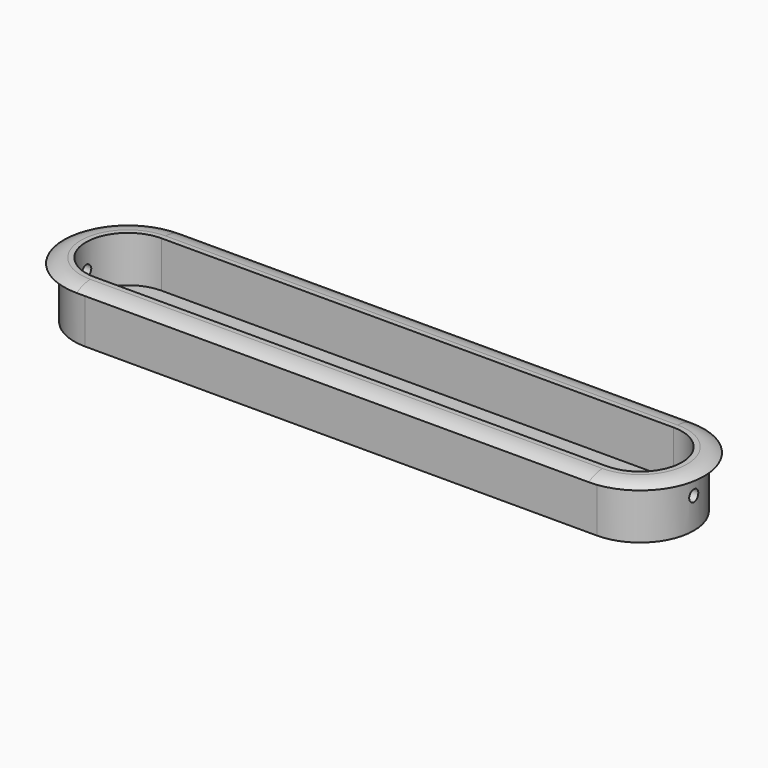
from build123d import *

# Parameters (mm, degrees)
F1_DEPTH    = 10
F3_DEPTH    = 1
F4_T1_DEPTH = 100
F4_T4_ANGLE = 180
F4_T6_ANGLE = 180
F6_DEPTH    = 9
F7_R        = 1.1168399156
F8_DEPTH    = 100


# Not quite as in the source:
# - a fillet or chamfer that OpenCascade refuses, or shapes differently, is made with other operations: its cross-section is extruded or revolved along the edge and cut away or added


with BuildPart() as f1:
    # F0 (on Top) → F1 (new body)
    with BuildSketch(Plane.XY):
        with BuildLine():
            Line((48.6515399069, 4.7592671573), (-51.3484600931, 4.7592671573))
            ThreePointArc((-51.3484600931, 4.7592671573), (-61.8484600931, -5.7407328427), (-51.3484600931, -16.2407328427))
            Line((-51.3484600931, -16.2407328427), (48.6515399069, -16.2407328427))
            ThreePointArc((48.6515399069, -16.2407328427), (59.1515399069, -5.7407328427), (48.6515399069, 4.7592671573))
        make_face()
    extrude(amount=F1_DEPTH)

    # F2 (on face) → F3 (join)
    with BuildSketch(Plane.XY.offset(10)):
        with BuildLine():
            Line((48.6515399069, 6.7592671573), (-51.3484600931, 6.7592671573))
            ThreePointArc((-51.3484600931, 6.7592671573), (-63.8484600931, -5.7407328427), (-51.3484600931, -18.2407328427))
            Line((-51.3484600931, -18.2407328427), (48.6515399069, -18.2407328427))
            ThreePointArc((48.6515399069, -18.2407328427), (61.1515399069, -5.7407328427), (48.6515399069, 6.7592671573))
        make_face()
        with BuildLine():
            Line((-51.3484600931, 4.7592671573), (48.6515399069, 4.7592671573))
            ThreePointArc((48.6515399069, 4.7592671573), (59.1515399069, -5.7407328427), (48.6515399069, -16.2407328427))
            Line((48.6515399069, -16.2407328427), (-51.3484600931, -16.2407328427))
            ThreePointArc((-51.3484600931, -16.2407328427), (-61.8484600931, -5.7407328427), (-51.3484600931, 4.7592671573))
        make_face(mode=Mode.SUBTRACT)
        with BuildLine():
            ThreePointArc((48.6515399069, -16.2407328427), (59.1515399069, -5.7407328427), (48.6515399069, 4.7592671573))
            Line((48.6515399069, 4.7592671573), (-51.3484600931, 4.7592671573))
            ThreePointArc((-51.3484600931, 4.7592671573), (-61.8484600931, -5.7407328427), (-51.3484600931, -16.2407328427))
            Line((-51.3484600931, -16.2407328427), (48.6515399069, -16.2407328427))
        make_face()
    extrude(amount=F3_DEPTH)

    # F4: fillet of radius 6 on 4 edges, made by hand

    # F4_s2 → F4_t1 (cut)
    with BuildSketch(Plane.YZ.offset(-51.3484600931)):
        with BuildLine():
            ThreePointArc((6.7592671573, 10), (5.1746931745, 10.7445626465), (3.4426423669, 11))
            Line((3.4426423669, 11), (6.7592671573, 11))
            Line((6.7592671573, 11), (6.7592671573, 10))
        make_face()
        with BuildLine():
            ThreePointArc((-18.2407328427, 10), (-16.6561588599, 10.7445626465), (-14.9241080524, 11))
            Line((-14.9241080524, 11), (-18.2407328427, 11))
            Line((-18.2407328427, 11), (-18.2407328427, 10))
        make_face()
    extrude(amount=F4_T1_DEPTH, mode=Mode.SUBTRACT)

    # F4_s3 → F4_t4 (revolve, cut)
    with BuildSketch(Plane.YZ.offset(48.6515399069)):
        with BuildLine():
            ThreePointArc((-18.2407328427, 10), (-16.6561588599, 10.7445626465), (-14.9241080524, 11))
            Line((-14.9241080524, 11), (-18.2407328427, 11))
            Line((-18.2407328427, 11), (-18.2407328427, 10))
        make_face()
    revolve(axis=Axis((48.6515399069, -5.7407328427, 11), (0, 0, 1)), revolution_arc=F4_T4_ANGLE, mode=Mode.SUBTRACT)

    # F4_s5 → F4_t6 (revolve, cut)
    with BuildSketch(Plane.YZ.offset(-51.3484600931)):
        with BuildLine():
            ThreePointArc((3.4426423669, 11), (5.1746931745, 10.7445626465), (6.7592671573, 10))
            Line((6.7592671573, 10), (6.7592671573, 11))
            Line((6.7592671573, 11), (3.4426423669, 11))
        make_face()
    revolve(axis=Axis((-51.3484600931, -5.7407328427, 11), (0, 0, 1)), revolution_arc=F4_T6_ANGLE, mode=Mode.SUBTRACT)

    # F5 (on face) → F6 (cut)
    with BuildSketch(Plane.XY.offset(11)):
        with BuildLine():
            Line((48.6515399069, 2.4426423669), (-51.3484600931, 2.4426423669))
            ThreePointArc((-51.3484600931, 2.4426423669), (-59.5318353028, -5.7407328427), (-51.3484600931, -13.9241080524))
            Line((-51.3484600931, -13.9241080524), (48.6515399069, -13.9241080524))
            ThreePointArc((48.6515399069, -13.9241080524), (56.8349151165, -5.7407328427), (48.6515399069, 2.4426423669))
        make_face()
    extrude(amount=-F6_DEPTH, mode=Mode.SUBTRACT)

    # F7 (on Right) → F8 (cut, symmetric)
    with BuildSketch(Plane.YZ):
        with Locations((-5.6874994189, 6)):
            Circle(F7_R)
    extrude(amount=F8_DEPTH, both=True, mode=Mode.SUBTRACT)


solid = f1.part
